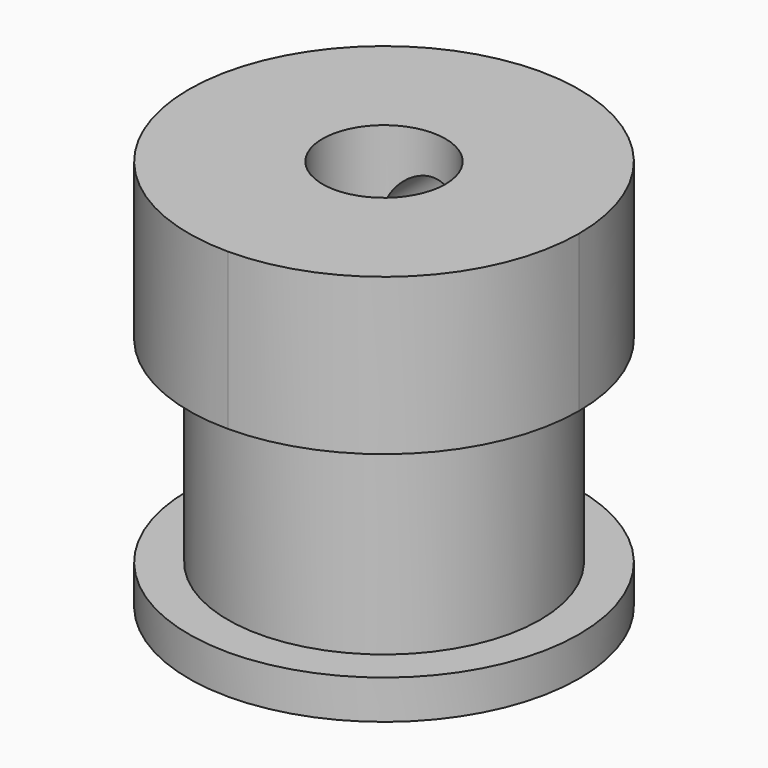
from build123d import *

# Parameters (mm, degrees)
F0_R         = 7.9375
F1_DEPTH     = 1.5875
F2_R         = 6.35
F3_DEPTH     = 8
F4_W         = 15.875
F4_H         = 15.875
F5_DEPTH     = 6.35
F6_R         = 2.5
F7_DEPTH     = 15.9375
F8_R         = 1.5875
F9_REACH     = 20.3661280605
F10_T1_DEPTH = 46.0375


# Not quite as in the source:
# - a fillet or chamfer that OpenCascade refuses, or shapes differently, is made with other operations: its cross-section is extruded or revolved along the edge and cut away or added


with BuildPart() as f1:
    # F0 (on Top) → F1 (new body)
    with BuildSketch(Plane.XY):
        Circle(F0_R)
    extrude(amount=F1_DEPTH)

    # F2 (on face) → F3 (join)
    with BuildSketch(Plane.XY.offset(1.5875)):
        Circle(F2_R)
    extrude(amount=F3_DEPTH)

    # F4 (on face) → F5 (join)
    with BuildSketch(Plane.XY.offset(9.5875)):
        Rectangle(F4_W, F4_H)
    extrude(amount=F5_DEPTH)

    # F6 (on face) → F7 (cut, through all)
    with BuildSketch(Plane.XY.offset(15.9375)):
        Circle(F6_R)
    extrude(amount=-F7_DEPTH, mode=Mode.SUBTRACT)

    f9_end = f1.faces().sort_by_distance((-2.5, 0, 7.96875))[0]
    # F8 (on face) → F9 (cut, up to a face of the model that its end follows)
    with BuildSketch(Plane(origin=(0, 7.9375, 0), x_dir=(-1, 0, 0), z_dir=(0, 1, 0))):
        with Locations((0, 12.7625)):
            Circle(F8_R)
    f9_long = extrude(amount=-F9_REACH, mode=Mode.PRIVATE)
    add(split(f9_long, bisect_by=f9_end, keep=Keep.ALL, mode=Mode.PRIVATE).solids().sort_by_distance((0, 7.9375, 12.7625))[0], mode=Mode.SUBTRACT)

    # F10: fillet of radius 7.9375 on 4 edges, made by hand

    # F10_s2 → F10_t1 (cut)
    with BuildSketch(Plane.XY.offset(-10.25625)):
        with BuildLine():
            ThreePointArc((-7.9375, 0), (-5.6126600757, 5.6126600757), (0, 7.9375))
            Line((0, 7.9375), (-7.9375, 7.9375))
            Line((-7.9375, 7.9375), (-7.9375, 0))
        make_face()
        with BuildLine():
            ThreePointArc((0, -7.9375), (-5.6126600757, -5.6126600757), (-7.9375, 0))
            Line((-7.9375, 0), (-7.9375, -7.9375))
            Line((-7.9375, -7.9375), (0, -7.9375))
        make_face()
        with BuildLine():
            ThreePointArc((7.9375, 0), (5.6126600757, 5.6126600757), (0, 7.9375))
            Line((0, 7.9375), (7.9375, 7.9375))
            Line((7.9375, 7.9375), (7.9375, 0))
        make_face()
        with BuildLine():
            ThreePointArc((0, -7.9375), (5.6126600757, -5.6126600757), (7.9375, 0))
            Line((7.9375, 0), (7.9375, -7.9375))
            Line((7.9375, -7.9375), (0, -7.9375))
        make_face()
    extrude(amount=F10_T1_DEPTH, mode=Mode.SUBTRACT)


solid = f1.part
